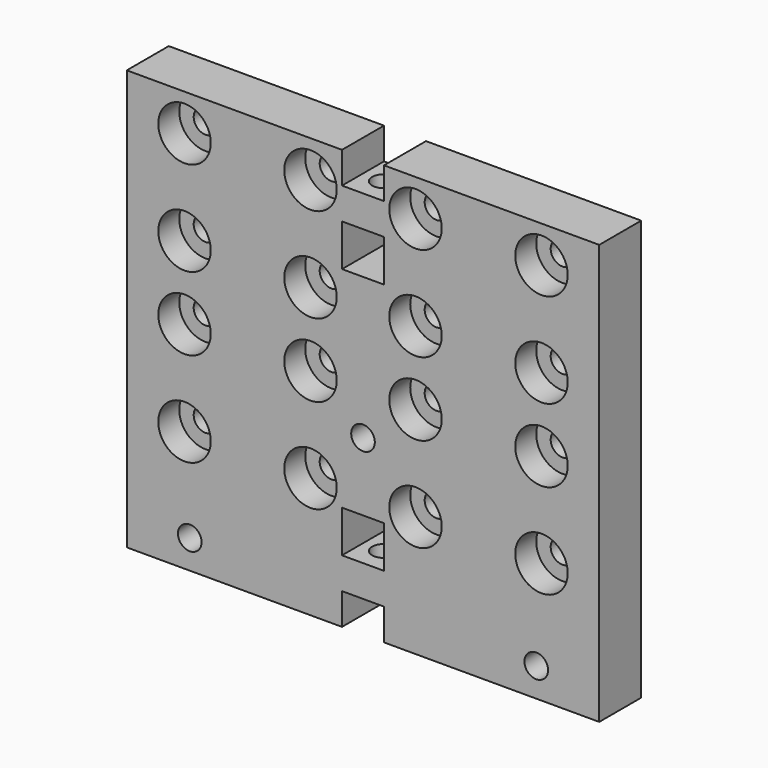
from build123d import *

# Parameters (mm, degrees)
F0_W      = 90
F0_H      = 80
F0_R      = 5
F0_R_2    = 2.25
F1_DEPTH  = 5
F2_DEPTH  = 10
F3_W      = 8
F3_H      = 8
F3_H_2    = 6
F4_DEPTH  = 10.001
F5_R      = 2.25
F6_DEPTH  = 20
F7_R      = 2.25
F8_DEPTH  = 20
F9_R      = 2.25
F10_DEPTH = 10.001


# Not quite as in the source:
# - a feature names something its author has since deleted; it is built from what else it names


with BuildPart() as f1:
    # F0 (on Front) → F1 (new body)
    with BuildSketch(Plane.XZ):
        with Locations((45, 40)):
            Rectangle(F0_W, F0_H)
        Polygon((40, 23), (40, 17), (6, 17), (6, 23), (6, 41), (6, 47), (40, 47), (40, 41), align=None, mode=Mode.SUBTRACT)
        Polygon((84, 23), (84, 17), (50, 17), (50, 23), (50, 41), (50, 47), (84, 47), (84, 41), align=None, mode=Mode.SUBTRACT)
        Polygon((6, 73), (6, 79), (40, 79), (40, 73), (40, 55), (40, 49), (6, 49), (6, 55), align=None, mode=Mode.SUBTRACT)
        Polygon((84, 55), (84, 49), (50, 49), (50, 55), (50, 73), (50, 79), (84, 79), (84, 73), align=None, mode=Mode.SUBTRACT)
        Polygon((40, 79), (6, 79), (6, 73), (6, 55), (6, 49), (40, 49), (40, 55), (40, 73), align=None)
        with BuildLine():
            ThreePointArc((16, 55), (11, 50), (6, 55))
            ThreePointArc((6, 55), (11, 60), (16, 55))
        make_face(mode=Mode.SUBTRACT)
        with Locations((35, 55)):
            Circle(F0_R, mode=Mode.SUBTRACT)
        with BuildLine():
            ThreePointArc((16, 73), (11, 68), (6, 73))
            ThreePointArc((6, 73), (11, 78), (16, 73))
        make_face(mode=Mode.SUBTRACT)
        with Locations((35, 73)):
            Circle(F0_R, mode=Mode.SUBTRACT)
        Polygon((50, 49), (84, 49), (84, 55), (84, 73), (84, 79), (50, 79), (50, 73), (50, 55), align=None)
        with BuildLine():
            ThreePointArc((60, 55), (55, 50), (50, 55))
            ThreePointArc((50, 55), (55, 60), (60, 55))
        make_face(mode=Mode.SUBTRACT)
        with Locations((79, 55)):
            Circle(F0_R, mode=Mode.SUBTRACT)
        with BuildLine():
            ThreePointArc((60, 73), (55, 68), (50, 73))
            ThreePointArc((50, 73), (55, 78), (60, 73))
        make_face(mode=Mode.SUBTRACT)
        with Locations((79, 73)):
            Circle(F0_R, mode=Mode.SUBTRACT)
        Polygon((6, 17), (40, 17), (40, 23), (40, 41), (40, 47), (6, 47), (6, 41), (6, 23), align=None)
        with BuildLine():
            ThreePointArc((16, 23), (11, 18), (6, 23))
            ThreePointArc((6, 23), (11, 28), (16, 23))
        make_face(mode=Mode.SUBTRACT)
        with Locations((35, 23)):
            Circle(F0_R, mode=Mode.SUBTRACT)
        with BuildLine():
            ThreePointArc((16, 41), (11, 36), (6, 41))
            ThreePointArc((6, 41), (11, 46), (16, 41))
        make_face(mode=Mode.SUBTRACT)
        with Locations((35, 41)):
            Circle(F0_R, mode=Mode.SUBTRACT)
        Polygon((50, 17), (84, 17), (84, 23), (84, 41), (84, 47), (50, 47), (50, 41), (50, 23), align=None)
        with BuildLine():
            ThreePointArc((60, 23), (55, 18), (50, 23))
            ThreePointArc((50, 23), (55, 28), (60, 23))
        make_face(mode=Mode.SUBTRACT)
        with Locations((79, 23)):
            Circle(F0_R, mode=Mode.SUBTRACT)
        with BuildLine():
            ThreePointArc((60, 41), (55, 36), (50, 41))
            ThreePointArc((50, 41), (55, 46), (60, 41))
        make_face(mode=Mode.SUBTRACT)
        with Locations((79, 41)):
            Circle(F0_R, mode=Mode.SUBTRACT)
        with Locations((79, 41)):
            Circle(F0_R)
        with Locations((79, 41)):
            Circle(F0_R_2, mode=Mode.SUBTRACT)
        with BuildLine():
            ThreePointArc((16, 23), (11, 28), (6, 23))
            ThreePointArc((6, 23), (11, 18), (16, 23))
        make_face()
        with Locations((11, 23)):
            Circle(F0_R_2, mode=Mode.SUBTRACT)
        with BuildLine():
            ThreePointArc((16, 73), (11, 78), (6, 73))
            ThreePointArc((6, 73), (11, 68), (16, 73))
        make_face()
        with Locations((11, 73)):
            Circle(F0_R_2, mode=Mode.SUBTRACT)
        with Locations((35, 73)):
            Circle(F0_R)
        with Locations((35, 73)):
            Circle(F0_R_2, mode=Mode.SUBTRACT)
        with BuildLine():
            ThreePointArc((60, 73), (55, 78), (50, 73))
            ThreePointArc((50, 73), (55, 68), (60, 73))
        make_face()
        with Locations((55, 73)):
            Circle(F0_R_2, mode=Mode.SUBTRACT)
        with Locations((79, 73)):
            Circle(F0_R)
        with Locations((79, 73)):
            Circle(F0_R_2, mode=Mode.SUBTRACT)
        with Locations((79, 55)):
            Circle(F0_R)
        with Locations((79, 55)):
            Circle(F0_R_2, mode=Mode.SUBTRACT)
        with BuildLine():
            ThreePointArc((60, 55), (55, 60), (50, 55))
            ThreePointArc((50, 55), (55, 50), (60, 55))
        make_face()
        with Locations((55, 55)):
            Circle(F0_R_2, mode=Mode.SUBTRACT)
        with Locations((35, 55)):
            Circle(F0_R)
        with Locations((35, 55)):
            Circle(F0_R_2, mode=Mode.SUBTRACT)
        with BuildLine():
            ThreePointArc((16, 55), (11, 60), (6, 55))
            ThreePointArc((6, 55), (11, 50), (16, 55))
        make_face()
        with Locations((11, 55)):
            Circle(F0_R_2, mode=Mode.SUBTRACT)
        with Locations((35, 41)):
            Circle(F0_R)
        with Locations((35, 41)):
            Circle(F0_R_2, mode=Mode.SUBTRACT)
        with Locations((35, 23)):
            Circle(F0_R)
        with Locations((35, 23)):
            Circle(F0_R_2, mode=Mode.SUBTRACT)
        with BuildLine():
            ThreePointArc((16, 41), (11, 46), (6, 41))
            ThreePointArc((6, 41), (11, 36), (16, 41))
        make_face()
        with Locations((11, 41)):
            Circle(F0_R_2, mode=Mode.SUBTRACT)
        with BuildLine():
            ThreePointArc((60, 23), (55, 28), (50, 23))
            ThreePointArc((50, 23), (55, 18), (60, 23))
        make_face()
        with Locations((55, 23)):
            Circle(F0_R_2, mode=Mode.SUBTRACT)
        with BuildLine():
            ThreePointArc((60, 41), (55, 46), (50, 41))
            ThreePointArc((50, 41), (55, 36), (60, 41))
        make_face()
        with Locations((55, 41)):
            Circle(F0_R_2, mode=Mode.SUBTRACT)
        with Locations((79, 23)):
            Circle(F0_R)
        with Locations((79, 23)):
            Circle(F0_R_2, mode=Mode.SUBTRACT)
    extrude(amount=F1_DEPTH)

    # F0 (on Front) → F2 (join)
    with BuildSketch(Plane.XZ):
        with Locations((45, 40)):
            Rectangle(F0_W, F0_H)
        Polygon((40, 23), (40, 17), (6, 17), (6, 23), (6, 41), (6, 47), (40, 47), (40, 41), align=None, mode=Mode.SUBTRACT)
        Polygon((84, 23), (84, 17), (50, 17), (50, 23), (50, 41), (50, 47), (84, 47), (84, 41), align=None, mode=Mode.SUBTRACT)
        Polygon((6, 73), (6, 79), (40, 79), (40, 73), (40, 55), (40, 49), (6, 49), (6, 55), align=None, mode=Mode.SUBTRACT)
        Polygon((84, 55), (84, 49), (50, 49), (50, 55), (50, 73), (50, 79), (84, 79), (84, 73), align=None, mode=Mode.SUBTRACT)
        Polygon((50, 49), (84, 49), (84, 55), (84, 73), (84, 79), (50, 79), (50, 73), (50, 55), align=None)
        with BuildLine():
            ThreePointArc((60, 55), (55, 50), (50, 55))
            ThreePointArc((50, 55), (55, 60), (60, 55))
        make_face(mode=Mode.SUBTRACT)
        with Locations((79, 55)):
            Circle(F0_R, mode=Mode.SUBTRACT)
        with BuildLine():
            ThreePointArc((60, 73), (55, 68), (50, 73))
            ThreePointArc((50, 73), (55, 78), (60, 73))
        make_face(mode=Mode.SUBTRACT)
        with Locations((79, 73)):
            Circle(F0_R, mode=Mode.SUBTRACT)
        Polygon((50, 17), (84, 17), (84, 23), (84, 41), (84, 47), (50, 47), (50, 41), (50, 23), align=None)
        with BuildLine():
            ThreePointArc((60, 23), (55, 18), (50, 23))
            ThreePointArc((50, 23), (55, 28), (60, 23))
        make_face(mode=Mode.SUBTRACT)
        with Locations((79, 23)):
            Circle(F0_R, mode=Mode.SUBTRACT)
        with BuildLine():
            ThreePointArc((60, 41), (55, 36), (50, 41))
            ThreePointArc((50, 41), (55, 46), (60, 41))
        make_face(mode=Mode.SUBTRACT)
        with Locations((79, 41)):
            Circle(F0_R, mode=Mode.SUBTRACT)
        Polygon((6, 17), (40, 17), (40, 23), (40, 41), (40, 47), (6, 47), (6, 41), (6, 23), align=None)
        with BuildLine():
            ThreePointArc((16, 23), (11, 18), (6, 23))
            ThreePointArc((6, 23), (11, 28), (16, 23))
        make_face(mode=Mode.SUBTRACT)
        with Locations((35, 23)):
            Circle(F0_R, mode=Mode.SUBTRACT)
        with BuildLine():
            ThreePointArc((16, 41), (11, 36), (6, 41))
            ThreePointArc((6, 41), (11, 46), (16, 41))
        make_face(mode=Mode.SUBTRACT)
        with Locations((35, 41)):
            Circle(F0_R, mode=Mode.SUBTRACT)
        Polygon((40, 79), (6, 79), (6, 73), (6, 55), (6, 49), (40, 49), (40, 55), (40, 73), align=None)
        with BuildLine():
            ThreePointArc((16, 55), (11, 50), (6, 55))
            ThreePointArc((6, 55), (11, 60), (16, 55))
        make_face(mode=Mode.SUBTRACT)
        with Locations((35, 55)):
            Circle(F0_R, mode=Mode.SUBTRACT)
        with BuildLine():
            ThreePointArc((16, 73), (11, 68), (6, 73))
            ThreePointArc((6, 73), (11, 78), (16, 73))
        make_face(mode=Mode.SUBTRACT)
        with Locations((35, 73)):
            Circle(F0_R, mode=Mode.SUBTRACT)
    extrude(amount=F2_DEPTH)

    # F3 (on face) → F4 (cut, through all)
    with BuildSketch(Plane.XZ.offset(10)):
        with Locations((45, 64)):
            Rectangle(F3_W, F3_H)
        with Locations((45, 77)):
            Rectangle(F3_W, F3_H_2)
        with Locations((45, 16)):
            Rectangle(F3_W, F3_H)
        with Locations((45, 3)):
            Rectangle(F3_W, F3_H_2)
    extrude(amount=-F4_DEPTH, mode=Mode.SUBTRACT)

    # F5 (on face) → F6 (cut)
    with BuildSketch(Plane.XY.offset(80)):
        with Locations((45, -5)):
            Circle(F5_R)
    extrude(amount=-F6_DEPTH, mode=Mode.SUBTRACT)

    # F7 (on face) → F8 (cut)
    with BuildSketch(Plane(origin=(0, 0, 0), x_dir=(1, 0, 0), z_dir=(0, 0, -1))):
        with Locations((45, 5)):
            Circle(F7_R)
    extrude(amount=-F8_DEPTH, mode=Mode.SUBTRACT)

    # F9 (on face) → F10 (cut, through all)
    with BuildSketch(Plane.XZ.offset(10)):
        with Locations((45, 33)):
            Circle(F9_R)
        with Locations((12, 5.5)):
            Circle(F9_R)
        with Locations((78, 5.5)):
            Circle(F9_R)
    extrude(amount=-F10_DEPTH, mode=Mode.SUBTRACT)


solid = f1.part
